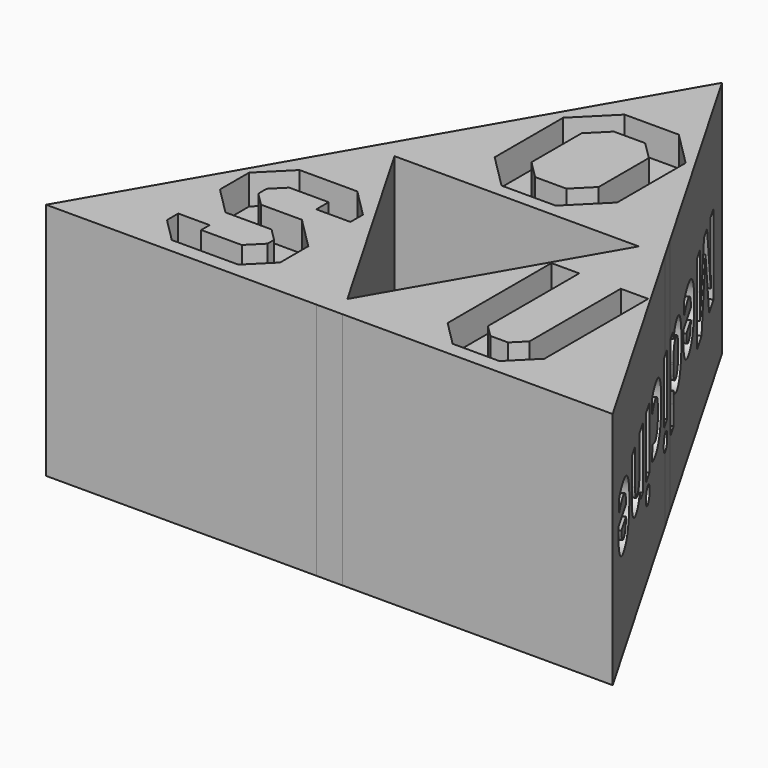
from build123d import *

# Parameters (mm, degrees)
F1_DEPTH     = 20.32
F2_SCALE     = 0.3
F5_TEXT_SIZE = 9.525
F6_DEPTH     = 0.762
F7_TEXT_SIZE = 9.525
F8_DEPTH     = 0.762
F9_W         = 2.3344060407
F9_H         = 7.9859190222
F10_DEPTH    = 2.54


# Not quite as in the source:
# - ends of sketch curves that miss each other by under 0.0002 mm in the source are joined
# - Text() gives the source's letters only with a copy of the font that has no kerning and outlines rounded to 1/6400 em; it was checked with that copy


with BuildPart() as f1:
    # F0 (on Top) → F1 (new body)
    with BuildSketch(Plane.XY):
        Polygon((24.4394496831, 42.9269748163), (12.9362464929, 23.0028424412), (35.938386165, 23.0028424412), (37.0462829749, 24.9217765051), (26.6509768831, 42.9269748163), align=None)
        Polygon((37.0462829749, 24.9217765051), (35.938386165, 23.0028429409), (38.1541800732, 23.0028424412), align=None)
        Polygon((25.5452132831, 44.8422135527), (24.4394496831, 42.9269748163), (26.6509768831, 42.9269748163), align=None)
        Polygon((37.0462829749, 24.9217765051), (38.1541800732, 23.0028424412), (61.160586165, 23.0028429409), (49.6573832634, 42.9269748163), (47.4415890666, 42.9269748163), align=None)
        Polygon((37.0484164732, 64.7663459278), (25.5452132831, 44.8422135527), (26.6509768831, 42.9269748163), (47.4415890666, 42.9269748163), (48.549486165, 44.8459088802), align=None)
        Polygon((48.549486165, 44.8459088802), (47.4415890666, 42.9269748163), (49.6573832634, 42.9269748163), align=None)
    extrude(amount=F1_DEPTH)


with BuildPart() as f1b:
    # F0 (on Top) → F1, piece 2 (new body)
    with BuildSketch(Plane.XY):
        Polygon((-27.0763959131, 14.4443714759), (-11.6844028517, 14.4443714759), (-2.004847629, 24.1239266985), (-2.004847629, 48.4059197599), (-11.6844028517, 58.0854749826), (-27.0763959131, 58.0854749826), (-36.7559511357, 48.4059197599), (-36.7559511357, 24.1239266985), align=None)
        Polygon((-28.9073512201, 27.3749232292), (-28.9073512201, 45.1549232292), (-23.8253993824, 50.2368750669), (-14.9353993824, 50.2368750669), (-9.8534475446, 45.1549232292), (-9.8534475446, 27.3749232292), (-14.9353993824, 22.2929713915), (-23.8253993824, 22.2929713915), align=None, mode=Mode.SUBTRACT)
    extrude(amount=F1_DEPTH)


with BuildPart() as f1b_1:
    # F2: moved
    add(f1b.part.scale(F2_SCALE))


with BuildPart() as f1b_2:
    # F3: moved
    add(f1b_1.part.moved(Location((42.9768, 39.7256, 17.78))))


with BuildPart() as f1_1:
    add(f1.part)

    # F4: cut F1b
    add(f1b_2.part, mode=Mode.SUBTRACT)

    # F5 (on face) → F6 (cut)
    with BuildSketch(Plane(origin=(-0.258338087, 0.1491515641, 0), x_dir=(-0.5, -0.8660254038, 0), z_dir=(-0.8660254038, 0.5, 0))):
        with Locations(Location((-33.124061056, 12.9989160818), (0, 0, -180))):
            Text('Sports', F5_TEXT_SIZE, font='Open Sans', font_style=FontStyle.BOLD, text_align=(TextAlign.LEFT, TextAlign.BOTTOM))
    extrude(amount=-F6_DEPTH, mode=Mode.SUBTRACT)

    # F7 (on face) → F8 (cut)
    with BuildSketch(Plane(origin=(55.8309627968, 32.2340213998, 0), x_dir=(-0.5, 0.8660254038, 0), z_dir=(0.8660254038, 0.5, 0))):
        with Locations(Location((34.7309494391, 12.7873101644), (0, 0, 180))):
            Text('Medicine', F7_TEXT_SIZE, font='Open Sans', font_style=FontStyle.BOLD, text_align=(TextAlign.LEFT, TextAlign.BOTTOM))
    extrude(amount=-F8_DEPTH, mode=Mode.SUBTRACT)

    # F9 (on face) → F10 (cut)
    with BuildSketch(Plane.XY.offset(20.32)):
        Polygon((23.2583453397, 27.5018935677), (20.5858312547, 27.5018935677), (20.5858312547, 26.3022724539), (22.6365976967, 24.2515060119), (28.3050683327, 24.2515060119), (30.2791856229, 26.2256233021), (30.2791856229, 29.2193359378), (27.5664730612, 31.9320484996), (24.5804544538, 31.9320484996), (24.5804544538, 29.5847449452), (26.8626008183, 29.5847449452), (27.9282600245, 28.5190857389), (27.9282600245, 28.1596500427), (27.9282600245, 27.818887364), (26.7119947821, 26.6026221216), (24.5804544538, 26.6026221216), (23.2583453397, 26.6026221216), align=None)
        Polygon((24.5804544538, 37.4235094127), (22.9744531747, 37.4235094127), (20.5858312547, 35.0348874927), (20.5858312547, 33.8879004121), (20.5858312547, 31.9377102676), (22.9387965771, 29.5847449452), (24.5804544538, 29.5847449452), (24.5804544538, 31.9320484996), (24.0847188979, 31.9320484996), (22.950399667, 33.0663677305), (22.950399667, 33.950092271), (24.0208227187, 35.0205153227), (27.3722755753, 35.0205153227), (27.3722755753, 33.7045669524), (30.2791856229, 33.7045669524), (30.2791856229, 35.0348874927), (27.8905637029, 37.4235094127), align=None)
        Polygon((46.7776730657, 37.4235056874), (44.4112233818, 37.4235056874), (44.4112233818, 33.8879004121), (44.4112233818, 26.3789072633), (46.5386246331, 24.2515060119), (50.5203024485, 24.2515060119), (52.6477036998, 26.3789072633), (52.6477036998, 29.4375866652), (50.3132976592, 29.4375866652), (50.3132976592, 27.7178213), (49.2991171777, 26.7036408186), (47.7868914604, 26.7036408186), (46.7776730657, 27.7128592134), align=None)
        with Locations((51.4805006795, 33.4305461763)):
            Rectangle(F9_W, F9_H)
    extrude(amount=-F10_DEPTH, mode=Mode.SUBTRACT)


solid = f1_1.part
